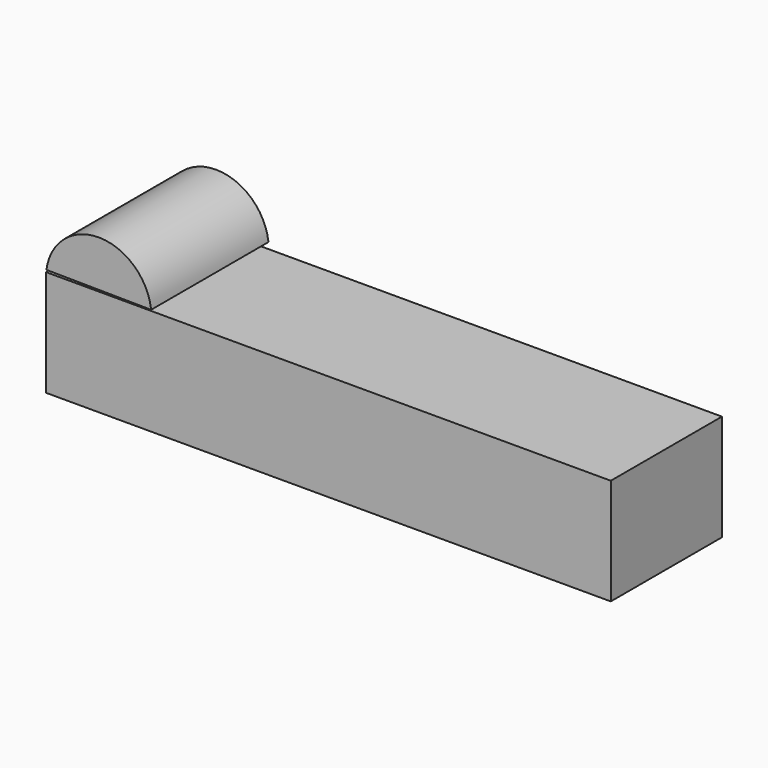
from build123d import *

# Parameters (mm, degrees)
F0_W     = 134.9828541279
F0_H     = 33.2014299929
F1_DEPTH = 25.4
F3_DEPTH = 16.51
F4_DEPTH = 18.542


# Not quite as in the source:
# - a feature of the source that left no trace in its solid (it failed there, or was rolled back) is left out


with BuildPart() as f1:
    # F0 (on Top) → F1 (new body)
    with BuildSketch(Plane.XY):
        Rectangle(F0_W, F0_H)
    extrude(amount=F1_DEPTH)


with BuildPart() as f3:
    # F2 (on Front) → F3 (new body)
    with BuildSketch(Plane.XZ):
        with BuildLine():
            Line((-67.4914270639, 25.8535724133), (-42.4542874098, 25.5814287812))
            ThreePointArc((-42.4542874098, 25.5814287812), (-54.8529271081, 36.7510396112), (-67.4914270639, 25.8535724133))
        make_face()
    extrude(amount=F3_DEPTH)

    # F4 (add): a face of the model
    f4_faces = [f3.faces().sort_by_distance(p)[0] for p in [
        (-54.9224588706, 0, 30.3541364957),
    ]]
    extrude(f4_faces, amount=F4_DEPTH)


solid = Compound([f1.part, f3.part])
